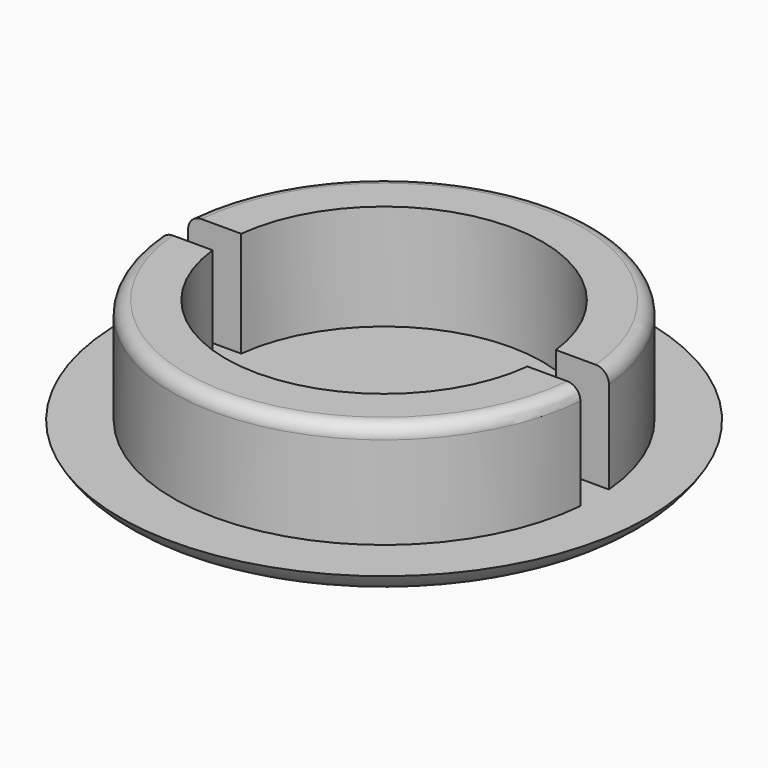
from build123d import *

# Parameters (mm, degrees)
F0_R     = 10
F1_DEPTH = 1
F3_R     = 8
F4_DEPTH = 4
F5_R     = 6
F6_DEPTH = 4
F7_W     = 17.3227433115
F7_H     = 1.3524350361
F8_DEPTH = 25
F9_R     = 0.5


# Not quite as in the source:
# - a fillet or chamfer that OpenCascade refuses, or shapes differently, is made with other operations: its cross-section is extruded or revolved along the edge and cut away or added


with BuildPart() as f1:
    # F0 (on Top) → F1 (new body)
    with BuildSketch(Plane.XY):
        Circle(F0_R)
    extrude(amount=F1_DEPTH)

    # F2: fillet of radius 2 on 1 edges, made by hand

    # F2_s1 → F2_t2 (revolve, cut)
    with BuildSketch(Plane.XZ):
        with BuildLine():
            ThreePointArc((10, 1), (9.2679491924, 0.2679491924), (8.2679491924, 0))
            Line((8.2679491924, 0), (10, 0))
            Line((10, 0), (10, 1))
        make_face()
    revolve(axis=Axis((0, 0, 0), (0, 0, 1)), mode=Mode.SUBTRACT)

    # F3 (on face) → F4 (join)
    with BuildSketch(Plane.XY.offset(1)):
        Circle(F3_R)
    extrude(amount=F4_DEPTH)

    # F5 (on face) → F6 (cut)
    with BuildSketch(Plane.XY.offset(5)):
        Circle(F5_R)
    extrude(amount=-F6_DEPTH, mode=Mode.SUBTRACT)

    # F7 (on face) → F8 (cut)
    with BuildSketch(Plane.XY.offset(1)):
        with Locations((-0.0975718722, 0.0086750078)):
            Rectangle(F7_W, F7_H)
    extrude(amount=F8_DEPTH, mode=Mode.SUBTRACT)

    # F9
    f9_edges = [f1.edges().sort_by_distance(p)[0] for p in [
        (0, 8, 5),
        (0, -8, 5),
    ]]
    fillet(f9_edges, radius=F9_R)


solid = f1.part
